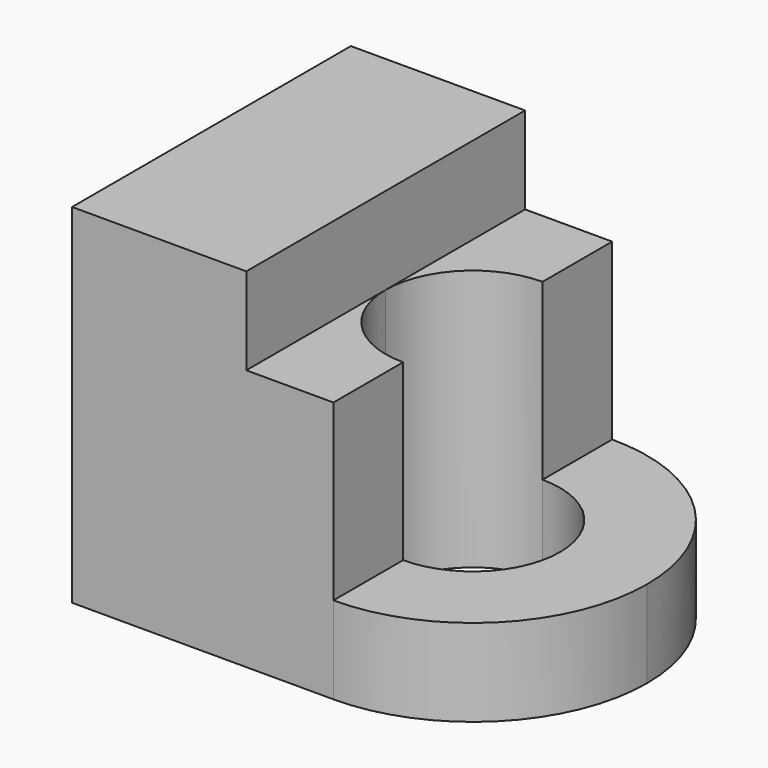
from build123d import *

# Parameters (mm, degrees)
F1_DEPTH = 20
F2_R     = 19.99999
F4_DEPTH = 30.001


# Not quite as in the source:
# - a fillet or chamfer is up to 0.001 mm smaller than in the source, because OpenCascade refuses the exact size


with BuildPart() as f1:
    # F0 (on Front) → F1 (new body, symmetric)
    with BuildSketch(Plane.XZ):
        Polygon((0, 40), (0, 0), (50, 0), (50, 10), (30, 10), (30, 30), (20, 30), (20, 40), align=None)
    extrude(amount=F1_DEPTH, both=True)

    # F2 (radius 20 in the source; OpenCascade refuses exactly that, so slightly less here)
    f2_edges = [f1.edges().sort_by_distance(p)[0] for p in [
        (50, -20, 5),
        (50, 20, 5),
    ]]
    fillet(f2_edges, radius=F2_R)

    # F3 (on face) → F4 (cut, through all)
    with BuildSketch(Plane.XY.offset(30)):
        with BuildLine():
            Line((30, -10), (30, 10))
            ThreePointArc((30, 10), (22.9289321778, 7.0710678016), (20, -2.91e-08))
            ThreePointArc((20, -2.91e-08), (22.9289321984, -7.0710678222), (30, -10))
        make_face()
        with BuildLine():
            ThreePointArc((30, -10), (37.0710678119, -7.0710678119), (40, 0))
            ThreePointArc((40, 0), (37.0710678119, 7.0710678119), (30, 10))
            Line((30, 10), (30, -10))
        make_face()
    extrude(amount=-F4_DEPTH, mode=Mode.SUBTRACT)


solid = f1.part
